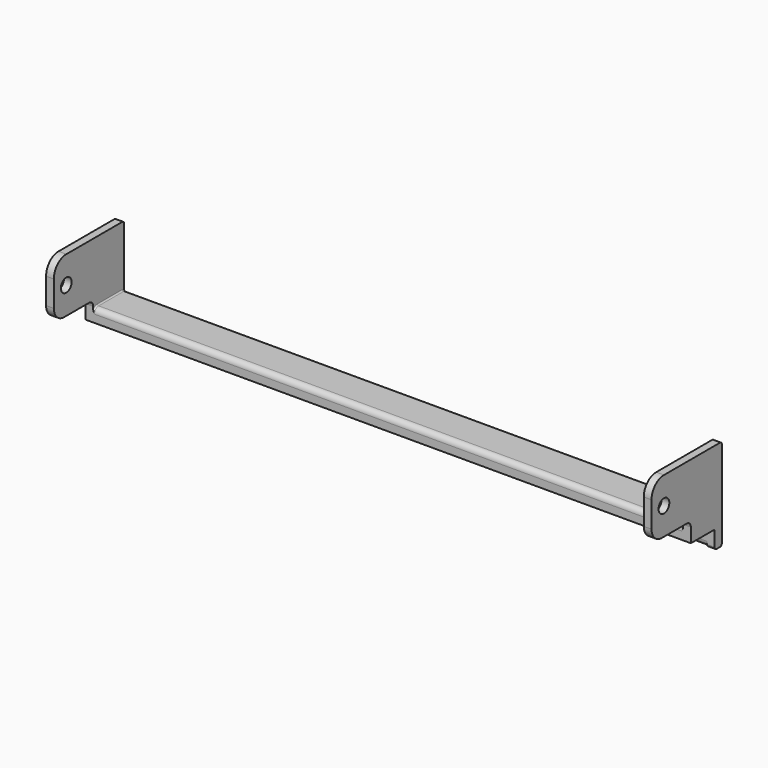
from build123d import *

# Parameters (mm, degrees)
F1_DEPTH     = 114
F3_DEPTH     = 3
F5_R         = 0.5
F6_D         = 5.2
F6_DEPTH     = 231.001
F7_D         = 5.2
F8_T1_DEPTH  = 12
F8_T6_ANGLE  = 161.6484946187
F8_T11_ANGLE = 150.9012204259
F8_T16_ANGLE = 150.9012204259
F8_T21_ANGLE = 161.6484946187


# Not quite as in the source:
# - a fillet or chamfer that OpenCascade refuses, or shapes differently, is made with other operations: its cross-section is extruded or revolved along the edge and cut away or added


with BuildPart() as f1:
    # F0 (on Right) → F1 (new body, symmetric)
    with BuildSketch(Plane.YZ):
        with BuildLine():
            Line((2.5, 5), (-9.5, 5))
            ThreePointArc((-9.5, 5), (-10.9142135624, 4.4142135624), (-11.5, 3))
            Line((-11.5, 3), (-11.5, 0))
            Line((-11.5, 0), (0, 0))
            Line((0, 0), (3.5, 0))
            Line((3.5, 0), (3.5, 4))
            ThreePointArc((3.5, 4), (3.2071067812, 4.7071067812), (2.5, 5))
        make_face()
        with BuildLine():
            Line((3.5, -6), (3.5, 0))
            Line((3.5, 0), (0, 0))
            Line((0, 0), (0, -5))
            ThreePointArc((0, -5), (0.5857864376, -6.4142135624), (2, -7))
            Line((2, -7), (2.5, -7))
            ThreePointArc((2.5, -7), (3.2071067812, -6.7071067812), (3.5, -6))
        make_face()
    extrude(amount=F1_DEPTH, both=True)

    # F2 (on face) → F3 (join)
    with BuildSketch(Plane.YZ.offset(114)):
        with BuildLine():
            Line((2.5, 28.5), (-24.5, 28.5))
            ThreePointArc((-24.5, 28.5), (-28.7426406871, 26.7426406871), (-30.5, 22.5))
            Line((-30.5, 22.5), (-30.5, 12.5))
            ThreePointArc((-30.5, 12.5), (-29.0355339059, 8.9644660941), (-25.5, 7.5))
            Line((-25.5, 7.5), (-13.5, 7.5))
            ThreePointArc((-13.5, 7.5), (-12.0857864376, 6.9142135624), (-11.5, 5.5))
            Line((-11.5, 5.5), (-11.5, 0))
            Line((-11.5, 0), (0, 0))
            Line((0, 0), (0, -6))
            ThreePointArc((0, -6), (0.2928932188, -6.7071067812), (1, -7))
            Line((1, -7), (2.5, -7))
            ThreePointArc((2.5, -7), (3.2071067812, -6.7071067812), (3.5, -6))
            Line((3.5, -6), (3.5, 7.5))
            Line((3.5, 7.5), (3.5, 27.5))
            ThreePointArc((3.5, 27.5), (3.2071067812, 28.2071067812), (2.5, 28.5))
        make_face()
    extrude(amount=F3_DEPTH)

    # F4: F1 across plane


with BuildPart() as f1_1:
    add(f1.part)
    add(f1.part.mirror(Plane.YZ))

    # F5
    f5_edges = [f1_1.edges().sort_by_distance(p)[0] for p in [
        (0, 0, 0),
    ]]
    fillet(f5_edges, radius=F5_R)

    # F6 (through all, one way)
    with BuildSketch(Plane.YZ.offset(114)):
        with Locations((-24.5, 18)):
            Circle(F6_D / 2)
    extrude(amount=-F6_DEPTH, mode=Mode.SUBTRACT)

    # F7 (through all)
    with Locations(Plane(origin=(114, 0, 0), x_dir=(0, 1, 0), z_dir=(-1, 0, 0))):
        with Locations((-24.5, -18)):
            Hole(F7_D / 2)

    # F8: fillet of radius 0.5 on 6 edges, made by hand

    # F8_s2 → F8_t1 (join)
    with BuildSketch(Plane.XZ.offset(-2.5)):
        with BuildLine():
            ThreePointArc((-114, 5.5), (-113.8535533906, 5.1464466094), (-113.5, 5))
            Line((-113.5, 5), (-114, 5))
            Line((-114, 5), (-114, 5.5))
        make_face()
        with BuildLine():
            ThreePointArc((114, 5.5), (113.8535533906, 5.1464466094), (113.5, 5))
            Line((113.5, 5), (114, 5))
            Line((114, 5), (114, 5.5))
        make_face()
    extrude(amount=F8_T1_DEPTH)


with BuildPart() as f8_tool4:
    # F8_s5 → F8_t6 (revolve)
    with BuildSketch(Plane(origin=(0, 3.4475148544, 1.1435956184), x_dir=(1, 0, 0), z_dir=(0, -0.9491428342, -0.3148458041))):
        with BuildLine():
            ThreePointArc((-114, 1.5094568264), (-113.8535533906, 1.863010217), (-113.5, 2.0094568264))
            Line((-113.5, 2.0094568264), (-114, 2.0094568264))
            Line((-114, 2.0094568264), (-114, 1.5094568264))
        make_face()
    revolve(axis=Axis((-114, 2.5, 4), (1, 0, 0)), revolution_arc=F8_T6_ANGLE)

    split(bisect_by=Plane.XZ.offset(-3.5), keep=Keep.TOP)


with BuildPart() as f1_2:
    add(f1_1.part)

    # F8_t3: union F8_tool4
    add(f8_tool4.part)


with BuildPart() as f8_tool9:
    # F8_s10 → F8_t11 (revolve)
    with BuildSketch(Plane.XZ.offset(9.5)):
        with BuildLine():
            ThreePointArc((-114, 5.5), (-113.8535533906, 5.1464466094), (-113.5, 5))
            Line((-113.5, 5), (-114, 5))
            Line((-114, 5), (-114, 5.5))
        make_face()
    revolve(axis=Axis((-114, -9.5, 3), (1, 0, 0)), revolution_arc=F8_T11_ANGLE)

    split(bisect_by=Plane.XZ.offset(11.5), keep=Keep.BOTTOM)


with BuildPart() as f1_3:
    add(f1_2.part)

    # F8_t8: union F8_tool9
    add(f8_tool9.part)


with BuildPart() as f8_tool14:
    # F8_s15 → F8_t16 (revolve)
    with BuildSketch(Plane.XZ.offset(9.5)):
        with BuildLine():
            ThreePointArc((113.5, 5), (113.8535533906, 5.1464466094), (114, 5.5))
            Line((114, 5.5), (114, 5))
            Line((114, 5), (113.5, 5))
        make_face()
    revolve(axis=Axis((114, -9.5, 3), (1, 0, 0)), revolution_arc=F8_T16_ANGLE)

    split(bisect_by=Plane.XZ.offset(11.5), keep=Keep.BOTTOM)


with BuildPart() as f1_4:
    add(f1_3.part)

    # F8_t13: union F8_tool14
    add(f8_tool14.part)


with BuildPart() as f8_tool19:
    # F8_s20 → F8_t21 (revolve)
    with BuildSketch(Plane(origin=(0, 3.4475148544, 1.1435956184), x_dir=(1, 0, 0), z_dir=(0, -0.9491428342, -0.3148458041))):
        with BuildLine():
            ThreePointArc((114, 1.5094568264), (113.8535533906, 1.863010217), (113.5, 2.0094568264))
            Line((113.5, 2.0094568264), (114, 2.0094568264))
            Line((114, 2.0094568264), (114, 1.5094568264))
        make_face()
    revolve(axis=Axis((114, 2.5, 4), (1, 0, 0)), revolution_arc=F8_T21_ANGLE)

    split(bisect_by=Plane.XZ.offset(-3.5), keep=Keep.TOP)


with BuildPart() as f1_5:
    add(f1_4.part)

    # F8_t18: union F8_tool19
    add(f8_tool19.part)


solid = f1_5.part
